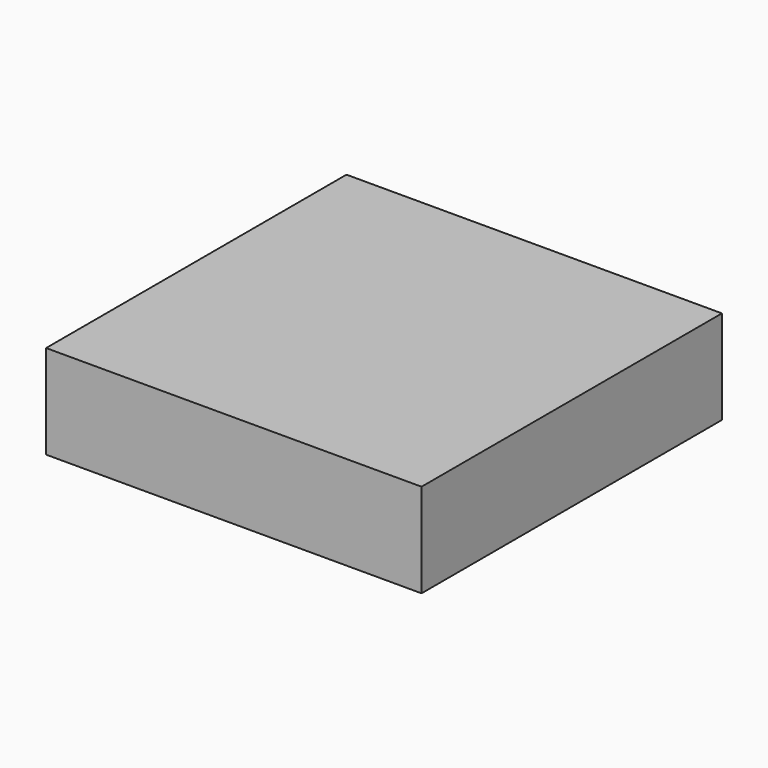
from build123d import *

# Parameters (mm, degrees)
F0_W     = 80
F0_H     = 80
F1_DEPTH = 20


# Not quite as in the source:
# - a feature names something its author has since deleted; it is built from what else it names


with BuildPart() as f1:
    # F0 (on Top) → F1 (new body)
    with BuildSketch(Plane.XY):
        Rectangle(F0_W, F0_H)
    extrude(amount=-F1_DEPTH)


solid = f1.part
